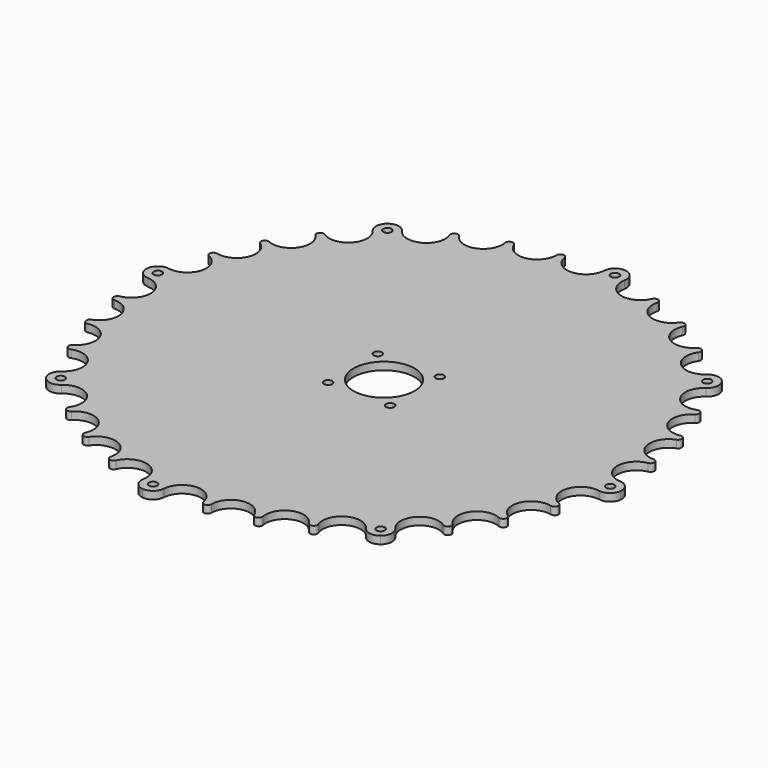
from build123d import *

# Parameters (mm, degrees)
F0_R            = 114.3
F0_R_2          = 1.7272
F0_R_3          = 12.7
F1_DEPTH        = 3.175
F2_R            = 1.7272
F3_DEPTH        = 3.175
F3_COPIES_COUNT = 8
F5_DEPTH        = 3.175
F5_COPIES_COUNT = 8


# Not quite as in the source:
# - a pattern or mirror of a feature is missing from the dataset's text; its kind, count and spacing are read off the source's solid


with BuildPart() as f1:
    # F0 (on Top) → F1 (new body)
    with BuildSketch(Plane.XY):
        Circle(F0_R)
        with Locations((-12.909118174, -12.909118174)):
            Circle(F0_R_2, mode=Mode.SUBTRACT)
        with Locations((12.909118174, -12.909118174)):
            Circle(F0_R_2, mode=Mode.SUBTRACT)
        with Locations((-12.909118174, 12.909118174)):
            Circle(F0_R_2, mode=Mode.SUBTRACT)
        Circle(F0_R_3, mode=Mode.SUBTRACT)
        with Locations((12.909118174, 12.909118174)):
            Circle(F0_R_2, mode=Mode.SUBTRACT)
    extrude(amount=F1_DEPTH)

    # F2 (on face) → F3 (cut, through all)
    with BuildSketch(Plane.XY.offset(3.175)):
        with Locations((-104.2084193553, 12.676744072)):
            Circle(F2_R)
    f3 = extrude(amount=-F3_DEPTH, mode=Mode.SUBTRACT)

    # F3_copies: F3 ×8 about axis
    f3_copies_axis = Axis((0, 0, 0), (0, 0, 1))
    for i in range(1, F3_COPIES_COUNT):
        add(f3.rotate(f3_copies_axis, i * 360 / F3_COPIES_COUNT), mode=Mode.SUBTRACT)

    # F4 (on face) → F5 (cut, through all)
    with BuildSketch(Plane.XY.offset(3.175)):
        with BuildLine():
            ThreePointArc((-86.3999070415, -67.6589569107), (-87.3583729083, -64.0047703869), (-85.3543905267, -60.8023040588))
            ThreePointArc((-85.3543905267, -60.8023040588), (-82.8464143249, -50.5540157704), (-92.7324291182, -46.8683585731))
            ThreePointArc((-92.7324291182, -46.8683585731), (-94.7342307933, -46.0827839435), (-94.1165439867, -44.0229780172))
            ThreePointArc((-94.1165439867, -44.0229780172), (-90.7433842392, -34.3836080304), (-99.6573570235, -29.3999598059))
            ThreePointArc((-99.6573570235, -29.3999598059), (-101.4849334974, -28.2666894598), (-100.5063583602, -26.3518191911))
            ThreePointArc((-100.5063583602, -26.3518191911), (-95.4522238114, -17.4776215154), (-103.3228234926, -10.9699859169))
            ThreePointArc((-103.3228234926, -10.9699859169), (-104.9164008036, -9.5260853666), (-103.6089432811, -7.8187798076))
            ThreePointArc((-103.6089432811, -7.8187798076), (-97.0517244749, 0.4468259777), (-104.4965013095, 7.922965045))
            ThreePointArc((-104.4965013095, 7.922965045), (-107.8674695554, 9.6283415588), (-108.9360674025, 13.2518529234))
            Line((-108.9360674025, 13.2518529234), (-113.463553135, 13.8026124328))
            ThreePointArc((-113.463553135, 13.8026124328), (-110.1086855289, -30.6686708402), (-89.9907686886, -70.47092699))
            Line((-89.9907686886, -70.47092699), (-86.3999070415, -67.6589569107))
        make_face()
    f5 = extrude(amount=-F5_DEPTH, mode=Mode.SUBTRACT)

    # F5_copies: F5 ×8 about axis
    f5_copies_axis = Axis((0, 0, 0), (0, 0, 1))
    for i in range(1, F5_COPIES_COUNT):
        add(f5.rotate(f5_copies_axis, i * 360 / F5_COPIES_COUNT), mode=Mode.SUBTRACT)


solid = f1.part
